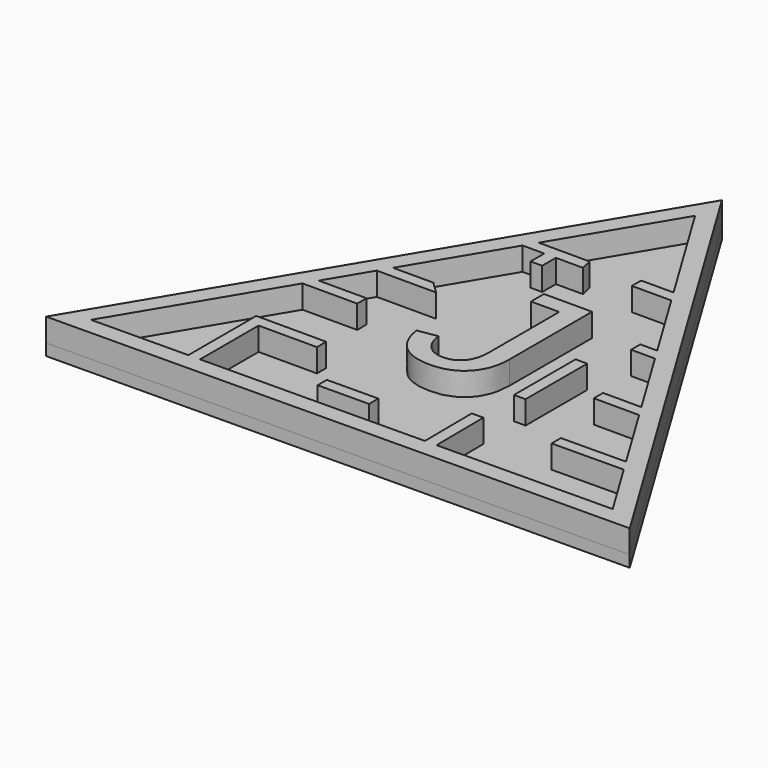
from build123d import *

# Parameters (mm, degrees)
F0_TEXT_SIZE = 36.8344519908
F0_W         = 2
F0_H         = 13.311563991
F1_DEPTH     = 6
F3_DEPTH     = 2


# Not quite as in the source:
# - Text() gives the source's letters only with a copy of the font that has no kerning and outlines rounded to 1/6400 em; it was checked with that copy


with BuildPart() as f1:
    # F0 (on Top) → F1 (new body)
    with BuildSketch(Plane.XY):
        Polygon((-49.8874282114, -34.8352881926), (50.1086562986, -33.9503686065), (0, 48.5685233198), align=None)
        Polygon((11.2247865867, 23.4646030217), (6.1445850879, 23.4646030217), (6.1445850879, 21.4646030217), (12.9487533615, 21.4646030217), (20.6074592748, 8.8522527367), (17.7000798285, 8.8522527367), (17.7000798285, 6.8522527367), (20.9371824382, 6.8522527367), (21.8219364721, 6.8522527367), (29.2348469285, -5.3553218022), (22.6253718138, -5.3553218022), (22.6253718138, -7.3553218022), (29.564570092, -7.3553218022), (30.4493241259, -7.3553218022), (37.5715882527, -19.0842602166), (26.405666766, -19.1830735119), (26.4233651577, -21.182995202), (38.7796212964, -21.0736479899), (44.8055735709, -30.9971809925), (14.6314238621, -31.2642084086), (14.5410370609, -21.0504823723), (12.5411637531, -21.0736479899), (12.6315021719, -31.2819068004), (-25.8933994959, -31.6228345497), (-25.8933994959, -18.9945939928), (-15.8297978342, -18.9945939928), (-15.8297978342, -16.9945939928), (-25.4909489304, -16.9945939928), (-27.9110985806, -16.9945939928), (-27.8933994959, -18.9945939928), (-27.8933994959, -31.6405336344), (-44.56906795, -31.7881056689), (-28.9565151544, -5.6864111684), (-28.1333792955, -5.6864111684), (-19.5226352662, -5.6864111684), (-19.5226352662, -3.6864111684), (-27.7602286225, -3.6864111684), (-23.4711264896, 3.4842825048), (-22.2748399577, 3.4842825048), (-13.2391210645, 3.4842825048), (-15.333625488, 5.4842825048), (-22.2748399577, 5.4842825048), (-12.7163188526, 21.4646030217), (-8.9696438569, 21.4646030217), (-8.9696438569, 18.5134038329), (-6.9696438569, 18.5134038329), (-6.9696438569, 21.4646030217), (-2.2955501557, 21.4646030217), (-2.7362388748, 23.4646030217), (-11.5200323207, 23.4646030217), (0.0193880345, 42.7566706784), (11.7342761641, 23.4646030217), align=None, mode=Mode.SUBTRACT)
        with Locations((-9.0101626702, -13.1221279153)):
            Text('J', F0_TEXT_SIZE, font='Arimo', text_align=(TextAlign.LEFT, TextAlign.BOTTOM))
        with Locations((14.6163033098, -6.6557819955)):
            Rectangle(F0_W, F0_H)
        Polygon((0, -25.5467354841), (-8.8207274675, -25.6247948855), (-8.8030290758, -27.6247165757), (0.0176983917, -27.5466571743), align=None)
    extrude(amount=F1_DEPTH)


with BuildPart() as f3:
    # F2 (on Top) → F3 (new body)
    with BuildSketch(Plane.XY):
        Polygon((-49.8874282114, -34.8352881926), (50.1086562986, -33.9503686065), (0, 48.5685233198), align=None)
    extrude(amount=F3_DEPTH)


solid = Compound([f1.part, f3.part])
